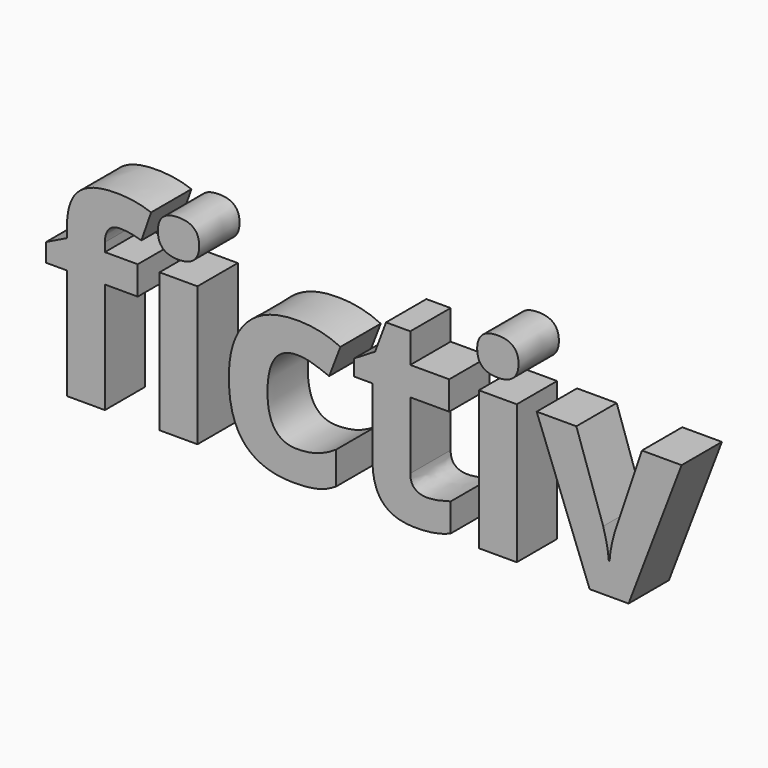
from build123d import *

# Parameters (mm, degrees)
F0_TEXT_SIZE = 202.1046665808
F1_DEPTH     = 40


# Not quite as in the source:
# - Text() gives the source's letters only with a copy of the font that has no kerning and outlines rounded to 1/6400 em; it was checked with that copy


with BuildPart() as f1:
    # F0 (on Front) → F1 (new body)
    with BuildSketch(Plane.XZ):
        with Locations((-264.7350425832, -72.9105249047)):
            Text('fictiv', F0_TEXT_SIZE, font='Open Sans', font_style=FontStyle.BOLD, text_align=(TextAlign.LEFT, TextAlign.BOTTOM))
    extrude(amount=F1_DEPTH)


solid = f1.part
